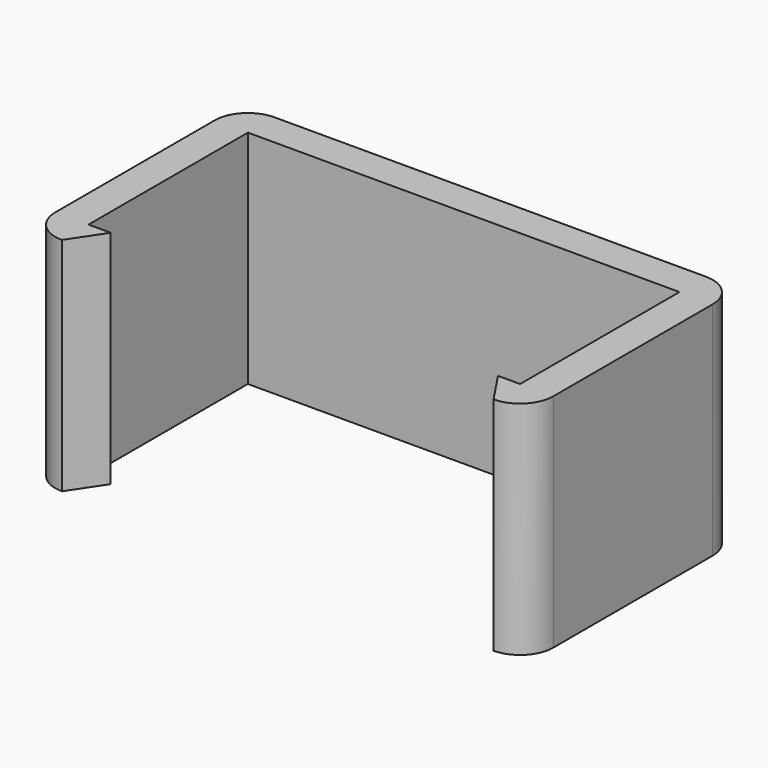
from build123d import *

# Parameters (mm, degrees)
F1_DEPTH = 20
F2_ANGLE = 270
F3_R     = 2.99999


# Not quite as in the source:
# - a fillet or chamfer is up to 0.001 mm smaller than in the source, because OpenCascade refuses the exact size


with BuildPart() as f1:
    # F0 (on Front) → F1 (new body)
    with BuildSketch(Plane.XZ):
        Polygon((22.5, 24), (-22.5, 24), (-22.5, 0), (-19.5, 0), (-17.5, 3), (-19.5, 3), (-19.5, 21), (19.5, 21), (19.5, 3), (17.5, 3), (19.5, 0), (22.5, 0), align=None)
    extrude(amount=F1_DEPTH)


with BuildPart() as f1_1:
    # F2: moved
    add(f1.part.rotate(Axis((0, -20, 24), (1, 0, 0)), F2_ANGLE))

    # F3 (radius 3 in the source; OpenCascade refuses exactly that, so slightly less here)
    f3_edges = [f1_1.edges().sort_by_distance(p)[0] for p in [
        (-22.5, -20, 14),
        (-22.5, -44, 14),
        (22.5, -44, 14),
        (22.5, -20, 14),
    ]]
    fillet(f3_edges, radius=F3_R)


solid = f1_1.part
